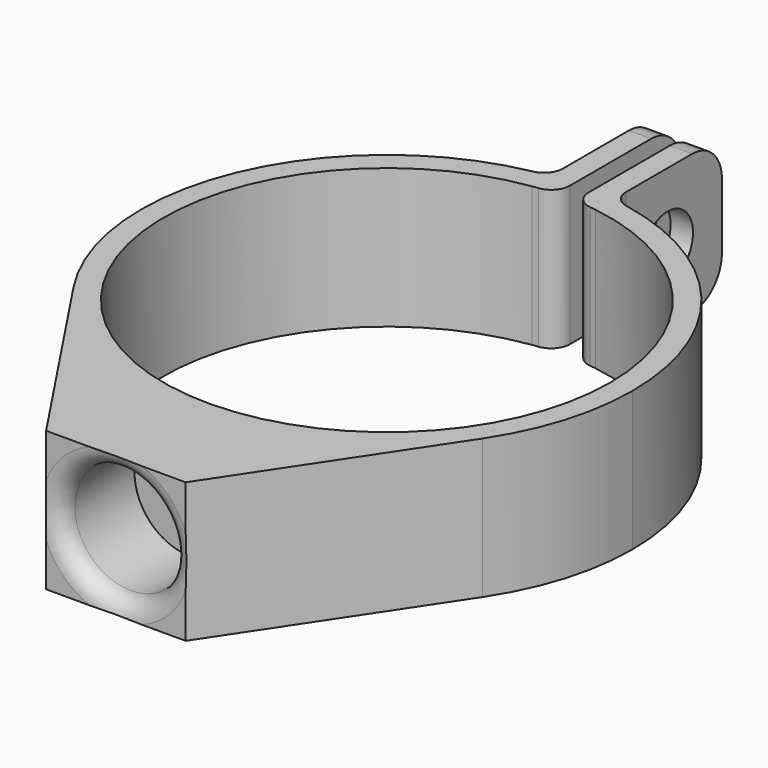
from build123d import *

# Parameters (mm, degrees)
F1_DEPTH    = 7.5
F2_R        = 3
F3_DEPTH    = 5
F4_R        = 2
F5_DEPTH    = 1.2
F6_R        = 1.7
F7_DEPTH    = 1.2
F8_T1_DEPTH = 7.5
F8_T3_DEPTH = 12.1179638093
F9_R        = 2


# Not quite as in the source:
# - a fillet or chamfer that OpenCascade refuses, or shapes differently, is made with other operations: its cross-section is extruded or revolved along the edge and cut away or added


with BuildPart() as f1:
    # F0 (on Top) → F1 (new body)
    with BuildSketch(Plane.XY):
        with BuildLine():
            ThreePointArc((10.9918685576, -7.3088182167), (0, -13.1999999285), (-10.9918685576, -7.3088182167))
            Line((-10.9918685576, -7.3088182167), (-3.75, -18.1999999285))
            Line((-3.75, -18.1999999285), (3.75, -18.1999999285))
            Line((3.75, -18.1999999285), (10.9918685576, -7.3088182167))
        make_face()
        with BuildLine():
            ThreePointArc((1.7, 11.8789730196), (9.0664215653, 7.8612976028), (12, 0))
            ThreePointArc((12, 0), (-7.8612976028, -9.0664215653), (-1.7, 11.8789730196))
            Line((-1.7, 11.8789730196), (-1.7, 13.0900725022))
            ThreePointArc((-1.7, 13.0900725022), (-12.0124754947, 5.4717849557), (-10.9918685576, -7.3088182167))
            ThreePointArc((-10.9918685576, -7.3088182167), (0, -13.1999999285), (10.9918685576, -7.3088182167))
            ThreePointArc((10.9918685576, -7.3088182167), (12.6359143374, -3.8175472451), (13.1999999285, 0))
            ThreePointArc((13.1999999285, 0), (9.9166526104, 8.7120605552), (1.7, 13.0900725022))
            Line((1.7, 13.0900725022), (1.7, 11.8789730196))
        make_face()
        with BuildLine():
            ThreePointArc((0.5, 13.1905268322), (1.1011461157, 13.1539908523), (1.7, 13.0900725022))
            Line((1.7, 13.0900725022), (1.7, 20.3789730196))
            Line((1.7, 20.3789730196), (0.5, 20.3789730196))
            Line((0.5, 20.3789730196), (0.5, 13.1905268322))
        make_face()
        with BuildLine():
            Line((-1.7, 20.3789730196), (-1.7, 13.0900725022))
            ThreePointArc((-1.7, 13.0900725022), (-1.1011461157, 13.1539908523), (-0.5, 13.1905268322))
            Line((-0.5, 13.1905268322), (-0.5, 20.3789730196))
            Line((-0.5, 20.3789730196), (-1.7, 20.3789730196))
        make_face()
        with BuildLine():
            Line((-1.7, 13.0900725022), (-1.7, 11.8789730196))
            ThreePointArc((-1.7, 11.8789730196), (-1.1013893091, 11.9493490028), (-0.5, 11.9895788083))
            Line((-0.5, 11.9895788083), (-0.5, 13.1905268322))
            ThreePointArc((-0.5, 13.1905268322), (-1.1011461157, 13.1539908523), (-1.7, 13.0900725022))
        make_face()
        with BuildLine():
            ThreePointArc((0.5, 11.9895788083), (1.1013893091, 11.9493490028), (1.7, 11.8789730196))
            Line((1.7, 11.8789730196), (1.7, 13.0900725022))
            ThreePointArc((1.7, 13.0900725022), (1.1011461157, 13.1539908523), (0.5, 13.1905268322))
            Line((0.5, 13.1905268322), (0.5, 11.9895788083))
        make_face()
    extrude(amount=F1_DEPTH)

    # F2 (on face) → F3 (cut)
    with BuildSketch(Plane.XZ.offset(18.1999999285)):
        with Locations((0, 3.75)):
            Circle(F2_R)
    extrude(amount=-F3_DEPTH, mode=Mode.SUBTRACT)

    # F4 (on face) → F5 (cut, through all)
    with BuildSketch(Plane(origin=(-1.7, 0, 0), x_dir=(0, -1, 0), z_dir=(-1, 0, 0))):
        with Locations((-16.7345227609, 3.75)):
            Circle(F4_R)
    extrude(amount=-F5_DEPTH, mode=Mode.SUBTRACT)

    # F6 (on face) → F7 (cut, through all)
    with BuildSketch(Plane.YZ.offset(1.7)):
        with Locations((16.7345227609, 3.75)):
            Circle(F6_R)
    extrude(amount=-F7_DEPTH, mode=Mode.SUBTRACT)

    # F8: fillet of radius 1 on 5 edges, made by hand

    # F8_s2 → F8_t1 (join)
    with BuildSketch(Plane.XY):
        with BuildLine():
            ThreePointArc((-2.509859154, 12.9591899878), (-1.9285919219, 13.3046060392), (-1.7, 13.9409468103))
            Line((-1.7, 13.9409468103), (-1.7, 13.0900725022))
            ThreePointArc((-1.7, 13.0900725022), (-2.1059466, 13.0309242585), (-2.509859154, 12.9591899878))
        make_face()
        with BuildLine():
            ThreePointArc((2.509859154, 12.9591899878), (1.9285919219, 13.3046060392), (1.7, 13.9409468103))
            Line((1.7, 13.9409468103), (1.7, 13.0900725022))
            ThreePointArc((1.7, 13.0900725022), (2.1059466, 13.0309242585), (2.509859154, 12.9591899878))
        make_face()
    extrude(amount=F8_T1_DEPTH)

    # F8_s4 → F8_t3 (cut)
    with BuildSketch(Plane.XY.offset(-2.3089819047)):
        with BuildLine():
            ThreePointArc((-1.3846153846, 11.9198506801), (-0.7532120062, 12.2481093984), (-0.5, 12.9131715701))
            Line((-0.5, 12.9131715701), (-0.5, 11.9895788083))
            ThreePointArc((-0.5, 11.9895788083), (-0.9429524325, 11.9628943283), (-1.3846153846, 11.9198506801))
        make_face()
        with BuildLine():
            ThreePointArc((0.5, 12.9131715701), (0.7532120062, 12.2481093984), (1.3846153846, 11.9198506801))
            ThreePointArc((1.3846153846, 11.9198506801), (0.9429524325, 11.9628943283), (0.5, 11.9895788083))
            Line((0.5, 11.9895788083), (0.5, 12.9131715701))
        make_face()
    extrude(amount=F8_T3_DEPTH, mode=Mode.SUBTRACT)

    # F8_s5 → F8_t6 (revolve, cut)
    with BuildSketch(Plane.XY.offset(3.75)):
        with BuildLine():
            ThreePointArc((4, -18.1999999285), (3.2928932188, -17.9071067097), (3, -17.1999999285))
            Line((3, -17.1999999285), (3, -18.1999999285))
            Line((3, -18.1999999285), (4, -18.1999999285))
        make_face()
    revolve(axis=Axis((0, -18.1999999285, 3.75), (0, -1, 0)), mode=Mode.SUBTRACT)

    # F9
    f9_edges = [f1.edges().sort_by_distance(p)[0] for p in [
        (-1.1, 20.378973, 7.5),
        (1.1, 20.378973, 7.5),
        (1.1, 20.378973, 0),
        (-1.1, 20.378973, 0),
    ]]
    fillet(f9_edges, radius=F9_R)


solid = f1.part
